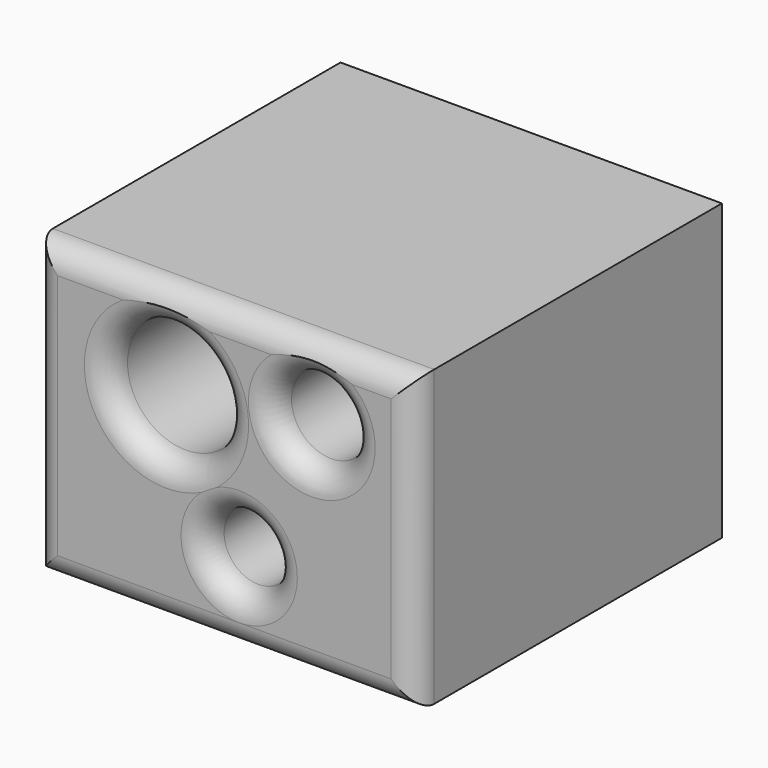
from build123d import *

# Parameters (mm, degrees)
F0_W        = 101.0252870619
F0_H        = 77.9844336212
F0_R        = 9.0586238997
F0_R_2      = 15.4013236799
F0_R_3      = 10.4395473454
F1_DEPTH    = 101.6
F2_T1_DEPTH = 132.7752870619
F2_T3_DEPTH = 109.7344336212


# Not quite as in the source:
# - a fillet or chamfer that OpenCascade refuses, or shapes differently, is made with other operations: its cross-section is extruded or revolved along the edge and cut away or added
# - a feature of the source that left no trace in its solid (it failed there, or was rolled back) is left out


with BuildPart() as f1:
    # F0 (on Front) → F1 (new body)
    with BuildSketch(Plane.XZ):
        with Locations((-15.3183694929, 6.5831001848)):
            Rectangle(F0_W, F0_H)
        with Locations((-11.3938301802, -10.6342416257)):
            Circle(F0_R, mode=Mode.SUBTRACT)
        with Locations((-30.6367408484, 20.7620896399)):
            Circle(F0_R_2, mode=Mode.SUBTRACT)
        with Locations((7.8490832821, 26.3324063271)):
            Circle(F0_R_3, mode=Mode.SUBTRACT)
    extrude(amount=F1_DEPTH)

    # F2: fillet of radius 6.35 on 7 edges, made by hand

    # F2_s2 → F2_t1 (cut)
    with BuildSketch(Plane.YZ.offset(-81.7060130239)):
        with BuildLine():
            ThreePointArc((-95.25, 45.5753169954), (-99.7401280605, 43.7154450559), (-101.6, 39.2253169954))
            Line((-101.6, 39.2253169954), (-101.6, 45.5753169954))
            Line((-101.6, 45.5753169954), (-95.25, 45.5753169954))
        make_face()
        with BuildLine():
            ThreePointArc((-95.25, -32.4091166258), (-99.7401280605, -30.5492446863), (-101.6, -26.0591166258))
            Line((-101.6, -26.0591166258), (-101.6, -32.4091166258))
            Line((-101.6, -32.4091166258), (-95.25, -32.4091166258))
        make_face()
    extrude(amount=F2_T1_DEPTH, mode=Mode.SUBTRACT)

    # F2_s4 → F2_t3 (cut)
    with BuildSketch(Plane.XY.offset(-48.2841166258)):
        with BuildLine():
            ThreePointArc((-65.8310130239, -95.25), (-63.9711410844, -99.7401280605), (-59.4810130239, -101.6))
            Line((-59.4810130239, -101.6), (-65.8310130239, -101.6))
            Line((-65.8310130239, -101.6), (-65.8310130239, -95.25))
        make_face()
        with BuildLine():
            ThreePointArc((35.1942740381, -95.25), (33.3344020986, -99.7401280605), (28.8442740381, -101.6))
            Line((28.8442740381, -101.6), (35.1942740381, -101.6))
            Line((35.1942740381, -101.6), (35.1942740381, -95.25))
        make_face()
    extrude(amount=F2_T3_DEPTH, mode=Mode.SUBTRACT)

    # F2_s5 → F2_t6 (revolve, cut)
    with BuildSketch(Plane.XY.offset(-10.6342416257)):
        with BuildLine():
            ThreePointArc((-2.3352062804, -95.25), (-0.475334341, -99.7401280605), (4.0147937196, -101.6))
            Line((4.0147937196, -101.6), (-2.3352062804, -101.6))
            Line((-2.3352062804, -101.6), (-2.3352062804, -95.25))
        make_face()
    revolve(axis=Axis((-11.3938301802, -101.6, -10.6342416257), (0, -1, 0)), mode=Mode.SUBTRACT)

    # F2_s7 → F2_t8 (revolve, cut)
    with BuildSketch(Plane.XY.offset(20.7620896399)):
        with BuildLine():
            ThreePointArc((-15.2354171685, -95.25), (-13.375545229, -99.7401280605), (-8.8854171685, -101.6))
            Line((-8.8854171685, -101.6), (-15.2354171685, -101.6))
            Line((-15.2354171685, -101.6), (-15.2354171685, -95.25))
        make_face()
    revolve(axis=Axis((-30.6367408484, -101.6, 20.7620896399), (0, -1, 0)), mode=Mode.SUBTRACT)

    # F2_s9 → F2_t10 (revolve, cut)
    with BuildSketch(Plane.XY.offset(26.3324063271)):
        with BuildLine():
            ThreePointArc((18.2886306275, -95.25), (20.1485025669, -99.7401280605), (24.6386306275, -101.6))
            Line((24.6386306275, -101.6), (18.2886306275, -101.6))
            Line((18.2886306275, -101.6), (18.2886306275, -95.25))
        make_face()
    revolve(axis=Axis((7.8490832821, -101.6, 26.3324063271), (0, -1, 0)), mode=Mode.SUBTRACT)


solid = f1.part
